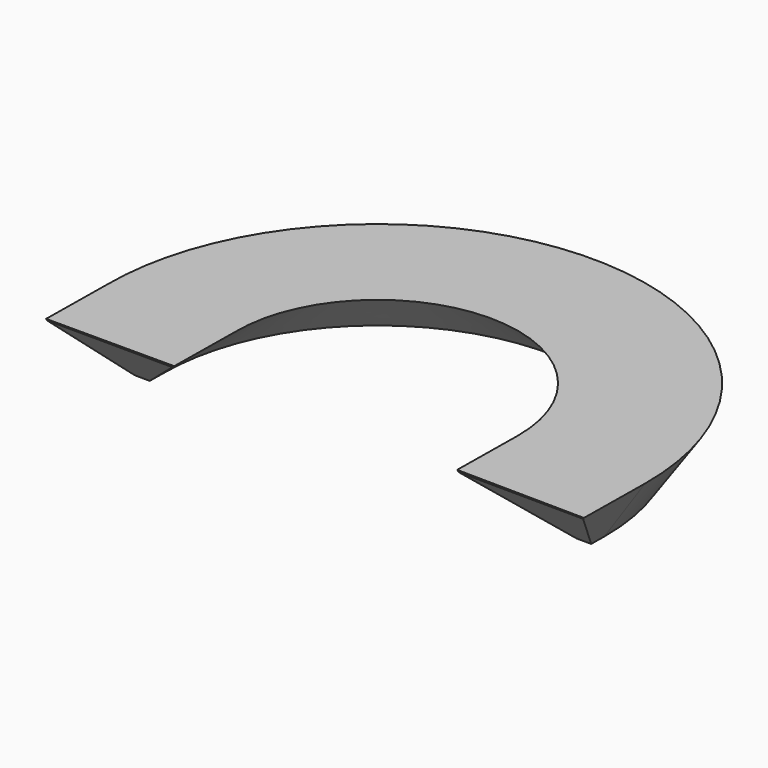
from build123d import *

# Parameters (mm, degrees)
F3_DEPTH = 1524
F4_SIZE  = 1193.8


# Not quite as in the source:
# - two fillets or chamfers of one size are made in one step


with BuildPart() as f2:
    # F2: sweep along a path in F0
    with BuildLine(Plane.XY) as f2_path:
        ThreePointArc((9143.8182811757, 0), (4571.9091405878, 4600.8237785405), (0, 0))
    # F1 (on Front) → F2 (sweep)
    with BuildSketch(Plane.XZ):
        Polygon((1715.5686188401, 0), (0, 0), (-879.0148030063, 0), (-47.9862770429, -1219.0467339141), (250.468130578, -1220.0421605104), align=None)
    sweep(path=f2_path.line)

    # F3 (add): faces of the model
    f3_faces = [f2.faces().sort_by_distance(p)[0] for p in [
        (8841.9781663596, 3.806076708, -448.4847642762),
        (301.8641103743, 0, -448.4847642762),
    ]]
    extrude(f3_faces, amount=F3_DEPTH, dir=(-0.0126085764, -0.9999205087, 0))

    # F4
    f4_edges = [f2.edges().sort_by_distance(p)[0] for p in [
        (9023.369932, -1522.602351, -1219.544447),
        (82.025456, -1523.878855, -1219.544447),
    ]]
    chamfer(f4_edges, length=F4_SIZE)


solid = f2.part
